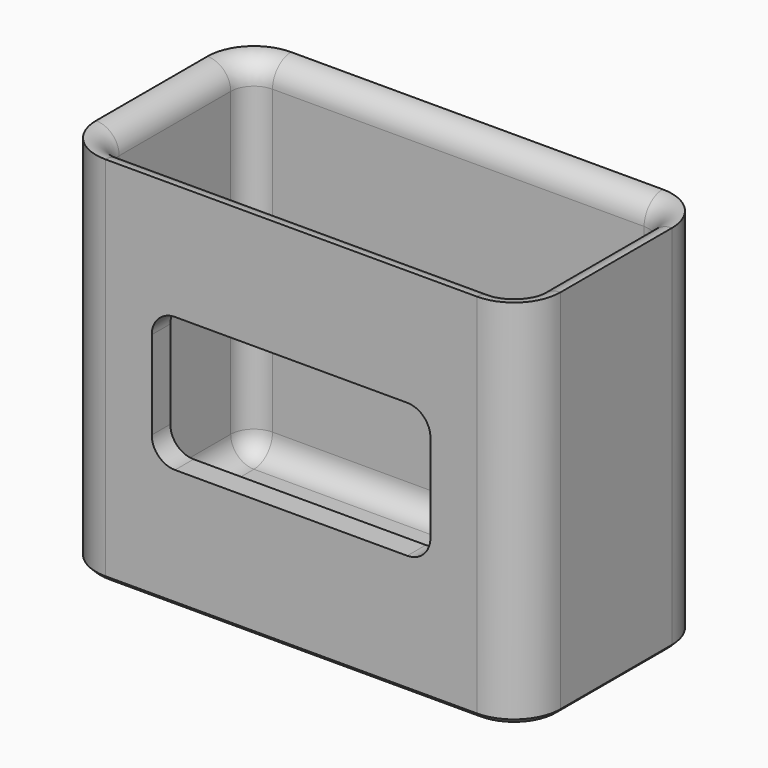
from build123d import *

# Parameters (mm, degrees)
F0_W     = 100
F0_H     = 50
F1_DEPTH = 80
F2_W     = 90
F2_H     = 40
F3_DEPTH = 75
F4_R     = 4.99999
F5_R     = 10
F6_SIZE  = 1
F8_DEPTH = 5


# Not quite as in the source:
# - a fillet or chamfer is up to 0.001 mm smaller than in the source, because OpenCascade refuses the exact size


with BuildPart() as f1:
    # F0 (on Top) → F1 (new body)
    with BuildSketch(Plane.XY):
        Rectangle(F0_W, F0_H)
    extrude(amount=F1_DEPTH)

    # F2 (on face) → F3 (cut)
    with BuildSketch(Plane.XY.offset(80)):
        Rectangle(F2_W, F2_H)
    extrude(amount=-F3_DEPTH, mode=Mode.SUBTRACT)

    # F4 (radius 5 in the source; OpenCascade refuses exactly that, so slightly less here)
    f4_edges = [f1.edges().sort_by_distance(p)[0] for p in [
        (45, 0, 5),
        (0, 20, 5),
        (0, -20, 5),
        (-45, 0, 5),
        (-45, 20, 42.5),
        (-45, -20, 42.5),
        (45, 20, 42.5),
        (45, -20, 42.5),
        (45, 0, 80),
        (0, 20, 80),
        (-45, 0, 80),
        (0, -20, 80),
    ]]
    fillet(f4_edges, radius=F4_R)

    # F5
    f5_edges = [f1.edges().sort_by_distance(p)[0] for p in [
        (50, -25, 40),
        (-50, -25, 40),
        (-50, 25, 40),
        (50, 25, 40),
    ]]
    fillet(f5_edges, radius=F5_R)

    # F6
    f6_edges = [f1.edges().sort_by_distance(p)[0] for p in [
        (0, -25, 0),
        (47.071068, -22.071068, 0),
        (50, 0, 0),
        (47.071068, 22.071068, 0),
        (0, 25, 0),
        (-47.071068, 22.071068, 0),
        (-50, 0, 0),
        (-47.071068, -22.071068, 0),
    ]]
    chamfer(f6_edges, length=F6_SIZE)

    # F7 (on face) → F8 (cut)
    with BuildSketch(Plane.XZ.offset(25)):
        with BuildLine():
            Line((25, 55), (-25, 55))
            ThreePointArc((-25, 55), (-28.5355339059, 53.5355339059), (-30, 50))
            Line((-30, 50), (-30, 31))
            ThreePointArc((-30, 31), (-28.5355339059, 27.4644660941), (-25, 26))
            Line((-25, 26), (25, 26))
            ThreePointArc((25, 26), (28.5355339059, 27.4644660941), (30, 31))
            Line((30, 31), (30, 50))
            ThreePointArc((30, 50), (28.5355339059, 53.5355339059), (25, 55))
        make_face()
    extrude(amount=-F8_DEPTH, mode=Mode.SUBTRACT)


solid = f1.part
